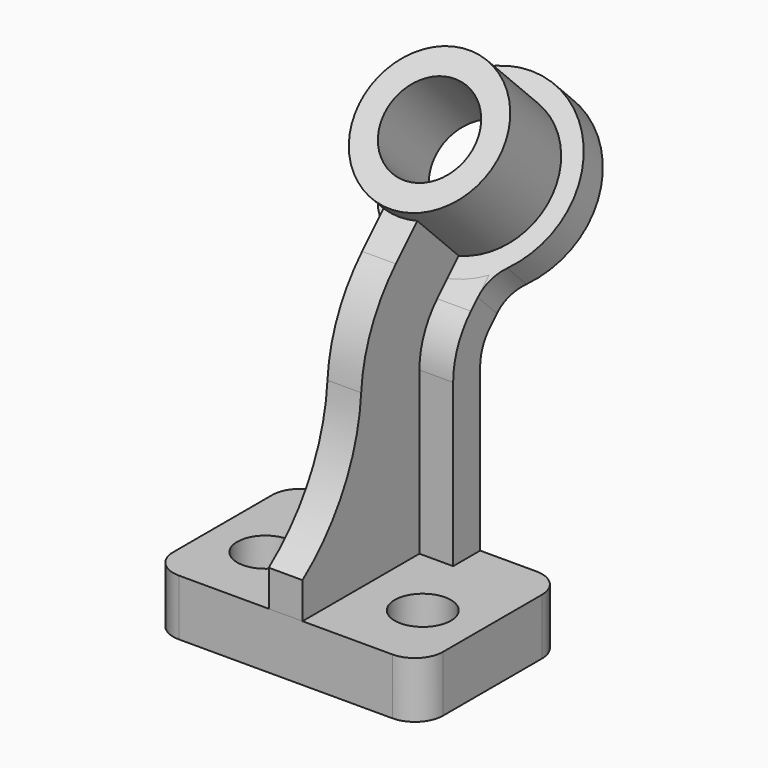
from build123d import *

# Parameters (mm, degrees)
F0_R           = 10
F1_DEPTH       = 20
F4_R           = 25
F4_R_2         = 16
F5_DEPTH       = 32
F6_R           = 32
F6_R_2         = 25
F7_DEPTH       = 12
F9_DEPTH       = 18
F9_DEPTH_BACK  = 18
F11_T1_DEPTH   = 12
F13_DEPTH      = 6
F13_DEPTH_BACK = 6


# Not quite as in the source:
# - a fillet or chamfer that OpenCascade refuses, or shapes differently, is made with other operations: its cross-section is extruded or revolved along the edge and cut away or added
# - the program builds the solid bodies; features that only make, move or delete a surface that nothing else refers to are left out


with BuildPart() as f1:
    # F0 (on Top) → F1 (new body)
    with BuildSketch(Plane.XY):
        with BuildLine():
            ThreePointArc((-48, 10), (-45.0710678119, 2.9289321881), (-38, 0))
            Line((-38, 0), (38, 0))
            ThreePointArc((38, 0), (45.0710678119, 2.9289321881), (48, 10))
            Line((48, 10), (48, 54))
            ThreePointArc((48, 54), (45.0710678119, 61.0710678119), (38, 64))
            Line((38, 64), (-38, 64))
            ThreePointArc((-38, 64), (-45.0710678119, 61.0710678119), (-48, 54))
            Line((-48, 54), (-48, 10))
        make_face()
        with Locations((-28, 26)):
            Circle(F0_R, mode=Mode.SUBTRACT)
        with Locations((28, 26)):
            Circle(F0_R, mode=Mode.SUBTRACT)
    extrude(amount=F1_DEPTH)


with BuildPart() as f5:
    # F4 (on face) → F5 (new body)
    with BuildSketch(Plane(origin=(0, -41, 41), x_dir=(-1, 0, 0), z_dir=(0, 0.7071067812, -0.7071067812))):
        with Locations((0, 148.4924240492)):
            Circle(F4_R)
        with Locations((0, 148.4924240492)):
            Circle(F4_R_2, mode=Mode.SUBTRACT)
    extrude(amount=F5_DEPTH)

    # F12 (on Right) → F13 (join, two sides)
    with BuildSketch(Plane.YZ) as f13_sk:
        with BuildLine():
            Line((52.0598683189, 125.5745869447), (41.5233405971, 115.0380592229))
            ThreePointArc((41.5233405971, 115.0380592229), (30.7052427168, 99.392946237), (26.1075371191, 80.9359176211))
            ThreePointArc((26.1075371191, 80.9359176211), (18.3506426226, 54.0218220938), (0, 32.8607288891))
            Line((0, 32.8607288891), (0, 20))
            Line((0, 20), (10, 20))
            Line((10, 20), (52, 20))
            Line((52, 20), (52, 77.56139982))
            ThreePointArc((52, 77.56139982), (54.0552526222, 87.8938524938), (59.908116908, 96.653282912))
            Line((59.908116908, 96.653282912), (62.9630978656, 99.7082638696))
            Line((62.9630978656, 99.7082638696), (70.5155401419, 107.2607061459))
            Line((70.5155401419, 107.2607061459), (52.0598683189, 125.5745869447))
        make_face()
    extrude(amount=F13_DEPTH)
    extrude(f13_sk.sketch, amount=-F13_DEPTH_BACK)


with BuildPart() as f7:
    # F6 (on face) → F7 (new body)
    with BuildSketch(Plane(origin=(0, -18.372583002, 18.372583002), x_dir=(-1, 0, 0), z_dir=(0, 0.7071067812, -0.7071067812))):
        with Locations((0, 148.4924240492)):
            Circle(F6_R)
        with Locations((0, 148.4924240492)):
            Circle(F6_R_2, mode=Mode.SUBTRACT)
    extrude(amount=F7_DEPTH)

    # F8 (on Right) → F9 (join, two sides)
    with BuildSketch(Plane.YZ) as f9_sk:
        with BuildLine():
            Line((52, 20), (64, 20))
            Line((64, 20), (64, 77.56139982))
            ThreePointArc((64, 77.56139982), (65.1418070123, 83.3016513055), (68.3933982822, 88.1680015378))
            Line((68.3933982822, 88.1680015378), (76.4746504982, 96.2492537538))
            Line((76.4746504982, 96.2492537538), (67.989369124, 104.7345351281))
            Line((67.989369124, 104.7345351281), (59.908116908, 96.653282912))
            ThreePointArc((59.908116908, 96.653282912), (54.0552526222, 87.8938524938), (52, 77.56139982))
            Line((52, 77.56139982), (52, 20))
        make_face()
    extrude(amount=F9_DEPTH)
    extrude(f9_sk.sketch, amount=-F9_DEPTH_BACK)

    # F10: union 

    # F11: fillet of radius 15 on 2 edges, made by hand

    # F11_s2 → F11_t1 (join)
    with BuildSketch(Plane(origin=(0, -9.8873016278, 9.8873016278), x_dir=(1, 0, 0), z_dir=(0, -0.7071067812, 0.7071067812))):
        with BuildLine():
            ThreePointArc((22.4680851064, 125.706789284), (19.1620318796, 120.8148603752), (18, 115.0260229878))
            Line((18, 115.0260229878), (18, 122.0349109385))
            ThreePointArc((18, 122.0349109385), (20.3171639431, 123.7697047548), (22.4680851064, 125.706789284))
        make_face()
        with BuildLine():
            ThreePointArc((-22.4680851064, 125.706789284), (-19.1620318796, 120.8148603752), (-18, 115.0260229878))
            Line((-18, 115.0260229878), (-18, 122.0349109385))
            ThreePointArc((-18, 122.0349109385), (-20.3171639431, 123.7697047548), (-22.4680851064, 125.706789284))
        make_face()
    extrude(amount=F11_T1_DEPTH)


solid = Compound([f1.part, f5.part, f7.part])
